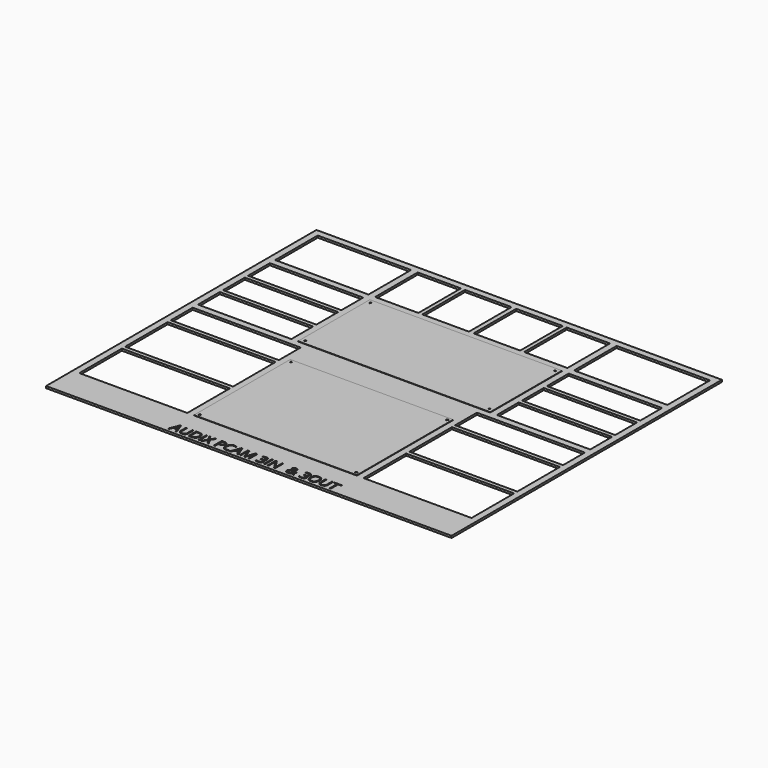
from build123d import *

# Parameters (mm, degrees)
F0_W         = 609.6
F0_H         = 508
F0_W_2       = 162.3
F0_H_2       = 80
F0_H_3       = 41
F0_W_3       = 245
F0_H_4       = 181
F0_W_4       = 140.3
F0_W_5       = 65
F0_W_6       = 70
F0_W_7       = 289
F0_H_5       = 135
F1_DEPTH     = 3
F0_R         = 1.4
F0_W_8       = 269
F0_H_6       = 115
F0_W_9       = 225
F0_H_7       = 161
F2_DEPTH     = 1.5
F3_TEXT_SIZE = 20.8333333333
F4_DEPTH     = 2
F5_SIZE2     = 0.692820323
F5_SIZE      = 0.4
F5_2_SIZE2   = 0.692820323
F5_2_SIZE    = 0.4
F5_3_SIZE2   = 0.692820323
F5_3_SIZE    = 0.4
F5_4_SIZE2   = 0.692820323
F5_4_SIZE    = 0.4
F5_5_SIZE2   = 0.692820323
F5_5_SIZE    = 0.4
F5_6_SIZE2   = 0.692820323
F5_6_SIZE    = 0.4
F5_7_SIZE2   = 0.692820323
F5_7_SIZE    = 0.4
F5_8_SIZE2   = 0.692820323
F5_8_SIZE    = 0.4
F6_START     = 2
F6_DEPTH     = 1.5


# Not quite as in the source:
# - Text() gives the source's letters only with a copy of the font that has no kerning and outlines rounded to 1/6400 em; it was checked with that copy


with BuildPart() as f1:
    # F0 (on Top) → F1 (new body)
    with BuildSketch(Plane.XY):
        Rectangle(F0_W, F0_H)
        with Locations((-213.65, -164)):
            Rectangle(F0_W_2, F0_H_2, mode=Mode.SUBTRACT)
        with Locations((-213.65, -78)):
            Rectangle(F0_W_2, F0_H_2, mode=Mode.SUBTRACT)
        with Locations((-213.65, -11.5)):
            Rectangle(F0_W_2, F0_H_3, mode=Mode.SUBTRACT)
        with Locations((213.65, -164)):
            Rectangle(F0_W_2, F0_H_2, mode=Mode.SUBTRACT)
        with Locations((0, -113.5)):
            Rectangle(F0_W_3, F0_H_4, mode=Mode.SUBTRACT)
        with Locations((213.65, -78)):
            Rectangle(F0_W_2, F0_H_2, mode=Mode.SUBTRACT)
        with Locations((213.65, -11.5)):
            Rectangle(F0_W_2, F0_H_3, mode=Mode.SUBTRACT)
        with Locations((-224.65, 39.5)):
            Rectangle(F0_W_4, F0_H_3, mode=Mode.SUBTRACT)
        with Locations((-224.65, 86.5)):
            Rectangle(F0_W_4, F0_H_3, mode=Mode.SUBTRACT)
        with Locations((-224.65, 133.5)):
            Rectangle(F0_W_4, F0_H_3, mode=Mode.SUBTRACT)
        with Locations((-224.65, 204)):
            Rectangle(F0_W_4, F0_H_2, mode=Mode.SUBTRACT)
        with Locations((-112, 204)):
            Rectangle(F0_W_5, F0_H_2, mode=Mode.SUBTRACT)
        with Locations((-38.5, 204)):
            Rectangle(F0_W_6, F0_H_2, mode=Mode.SUBTRACT)
        with Locations((0, 86.5)):
            Rectangle(F0_W_7, F0_H_5, mode=Mode.SUBTRACT)
        with Locations((224.65, 39.5)):
            Rectangle(F0_W_4, F0_H_3, mode=Mode.SUBTRACT)
        with Locations((224.65, 86.5)):
            Rectangle(F0_W_4, F0_H_3, mode=Mode.SUBTRACT)
        with Locations((38.5, 204)):
            Rectangle(F0_W_6, F0_H_2, mode=Mode.SUBTRACT)
        with Locations((112, 204)):
            Rectangle(F0_W_5, F0_H_2, mode=Mode.SUBTRACT)
        with Locations((224.65, 133.5)):
            Rectangle(F0_W_4, F0_H_3, mode=Mode.SUBTRACT)
        with Locations((224.65, 204)):
            Rectangle(F0_W_4, F0_H_2, mode=Mode.SUBTRACT)
    extrude(amount=F1_DEPTH)



with BuildPart() as f1b:
    # F0 (on Top) → F1, piece 2 (new body)
    with BuildSketch(Plane.XY):
        with Locations((-138.5, 148)):
            Circle(F0_R)
    extrude(amount=F1_DEPTH)


with BuildPart() as f1c:
    # F0 (on Top) → F1, piece 3 (new body)
    with BuildSketch(Plane.XY):
        with Locations((138.5, 148)):
            Circle(F0_R)
    extrude(amount=F1_DEPTH)


with BuildPart() as f1d:
    # F0 (on Top) → F1, piece 4 (new body)
    with BuildSketch(Plane.XY):
        with Locations((138.5, 25)):
            Circle(F0_R)
    extrude(amount=F1_DEPTH)


with BuildPart() as f1e:
    # F0 (on Top) → F1, piece 5 (new body)
    with BuildSketch(Plane.XY):
        with Locations((-138.5, 25)):
            Circle(F0_R)
    extrude(amount=F1_DEPTH)


with BuildPart() as f1f:
    # F0 (on Top) → F1, piece 6 (new body)
    with BuildSketch(Plane.XY):
        with Locations((-117.5, -28)):
            Circle(F0_R)
    extrude(amount=F1_DEPTH)


with BuildPart() as f1g:
    # F0 (on Top) → F1, piece 7 (new body)
    with BuildSketch(Plane.XY):
        with Locations((117.5, -28)):
            Circle(F0_R)
    extrude(amount=F1_DEPTH)


with BuildPart() as f1h:
    # F0 (on Top) → F1, piece 8 (new body)
    with BuildSketch(Plane.XY):
        with Locations((117.5, -199)):
            Circle(F0_R)
    extrude(amount=F1_DEPTH)


with BuildPart() as f1i:
    # F0 (on Top) → F1, piece 9 (new body)
    with BuildSketch(Plane.XY):
        with Locations((-117.5, -199)):
            Circle(F0_R)
    extrude(amount=F1_DEPTH)


with BuildPart() as f1_1:
    add(f1.part)

    add(f1b.part)  # F2 merges F1b

    add(f1c.part)  # F2 merges F1c

    add(f1d.part)  # F2 merges F1d

    add(f1e.part)  # F2 merges F1e

    add(f1f.part)  # F2 merges F1f

    add(f1g.part)  # F2 merges F1g

    add(f1h.part)  # F2 merges F1h

    add(f1i.part)  # F2 merges F1i
    # F0 (on Top) → F2 (join)
    with BuildSketch(Plane.XY):
        with Locations((0, 86.5)):
            Rectangle(F0_W_7, F0_H_5)
        with Locations((-138.5, 25)):
            Circle(F0_R, mode=Mode.SUBTRACT)
        with Locations((-138.5, 148)):
            Circle(F0_R, mode=Mode.SUBTRACT)
        with Locations((138.5, 25)):
            Circle(F0_R, mode=Mode.SUBTRACT)
        with Locations((0, 86.5)):
            Rectangle(F0_W_8, F0_H_6, mode=Mode.SUBTRACT)
        with Locations((138.5, 148)):
            Circle(F0_R, mode=Mode.SUBTRACT)
        with Locations((0, -113.5)):
            Rectangle(F0_W_3, F0_H_4)
        with Locations((-117.5, -199)):
            Circle(F0_R, mode=Mode.SUBTRACT)
        with Locations((-117.5, -28)):
            Circle(F0_R, mode=Mode.SUBTRACT)
        with Locations((117.5, -199)):
            Circle(F0_R, mode=Mode.SUBTRACT)
        with Locations((0, -113.5)):
            Rectangle(F0_W_9, F0_H_7, mode=Mode.SUBTRACT)
        with Locations((117.5, -28)):
            Circle(F0_R, mode=Mode.SUBTRACT)
    extrude(amount=F2_DEPTH)

    # F3 (on face) → F4 (cut)
    with BuildSketch(Plane.XY.offset(3)):
        with Locations((-125.3662109375, -249)):
            Text('AUDIX PCAM 3IN  & 3OUT', F3_TEXT_SIZE, font='Open Sans', text_align=(TextAlign.LEFT, TextAlign.BOTTOM))
    extrude(amount=-F4_DEPTH, mode=Mode.SUBTRACT)

    # F5
    f5_edges = [f1_1.edges().sort_by_distance(p)[0] for p in [
        (-139.9, 148, 3),
    ]]
    f5_side = f1_1.faces().sort_by_distance((-138.5, 148, 3))[0]
    chamfer(f5_edges, length=F5_SIZE, length2=F5_SIZE2, reference=f5_side)

    # F5#2
    f5_2_edges = [f1_1.edges().sort_by_distance(p)[0] for p in [
        (-139.9, 25, 3),
    ]]
    f5_2_side = f1_1.faces().sort_by_distance((-138.5, 25, 3))[0]
    chamfer(f5_2_edges, length=F5_2_SIZE, length2=F5_2_SIZE2, reference=f5_2_side)

    # F5#3
    f5_3_edges = [f1_1.edges().sort_by_distance(p)[0] for p in [
        (137.1, 25, 3),
    ]]
    f5_3_side = f1_1.faces().sort_by_distance((138.5, 25, 3))[0]
    chamfer(f5_3_edges, length=F5_3_SIZE, length2=F5_3_SIZE2, reference=f5_3_side)

    # F5#4
    f5_4_edges = [f1_1.edges().sort_by_distance(p)[0] for p in [
        (137.1, 148, 3),
    ]]
    f5_4_side = f1_1.faces().sort_by_distance((138.5, 148, 3))[0]
    chamfer(f5_4_edges, length=F5_4_SIZE, length2=F5_4_SIZE2, reference=f5_4_side)

    # F5#5
    f5_5_edges = [f1_1.edges().sort_by_distance(p)[0] for p in [
        (116.1, -28, 3),
    ]]
    f5_5_side = f1_1.faces().sort_by_distance((117.5, -28, 3))[0]
    chamfer(f5_5_edges, length=F5_5_SIZE, length2=F5_5_SIZE2, reference=f5_5_side)

    # F5#6
    f5_6_edges = [f1_1.edges().sort_by_distance(p)[0] for p in [
        (-118.9, -28, 3),
    ]]
    f5_6_side = f1_1.faces().sort_by_distance((-117.5, -28, 3))[0]
    chamfer(f5_6_edges, length=F5_6_SIZE, length2=F5_6_SIZE2, reference=f5_6_side)

    # F5#7
    f5_7_edges = [f1_1.edges().sort_by_distance(p)[0] for p in [
        (-118.9, -199, 3),
    ]]
    f5_7_side = f1_1.faces().sort_by_distance((-117.5, -199, 3))[0]
    chamfer(f5_7_edges, length=F5_7_SIZE, length2=F5_7_SIZE2, reference=f5_7_side)

    # F5#8
    f5_8_edges = [f1_1.edges().sort_by_distance(p)[0] for p in [
        (116.1, -199, 3),
    ]]
    f5_8_side = f1_1.faces().sort_by_distance((117.5, -199, 3))[0]
    chamfer(f5_8_edges, length=F5_8_SIZE, length2=F5_8_SIZE2, reference=f5_8_side)


with BuildPart() as f6:
    # F0 (on Top) → F6 (new body)
    with BuildSketch(Plane.XY.offset(F6_START)):
        with Locations((0, 86.5)):
            Rectangle(F0_W_7, F0_H_5)
        with Locations((-138.5, 25)):
            Circle(F0_R, mode=Mode.SUBTRACT)
        with Locations((-138.5, 148)):
            Circle(F0_R, mode=Mode.SUBTRACT)
        with Locations((138.5, 25)):
            Circle(F0_R, mode=Mode.SUBTRACT)
        with Locations((0, 86.5)):
            Rectangle(F0_W_8, F0_H_6, mode=Mode.SUBTRACT)
        with Locations((138.5, 148)):
            Circle(F0_R, mode=Mode.SUBTRACT)
        with Locations((0, 86.5)):
            Rectangle(F0_W_8, F0_H_6)
    extrude(amount=F6_DEPTH)


with BuildPart() as f6b:
    # F0 (on Top) → F6, piece 2 (new body)
    with BuildSketch(Plane.XY.offset(F6_START)):
        with Locations((0, -113.5)):
            Rectangle(F0_W_3, F0_H_4)
        with Locations((-117.5, -199)):
            Circle(F0_R, mode=Mode.SUBTRACT)
        with Locations((-117.5, -28)):
            Circle(F0_R, mode=Mode.SUBTRACT)
        with Locations((117.5, -199)):
            Circle(F0_R, mode=Mode.SUBTRACT)
        with Locations((0, -113.5)):
            Rectangle(F0_W_9, F0_H_7, mode=Mode.SUBTRACT)
        with Locations((117.5, -28)):
            Circle(F0_R, mode=Mode.SUBTRACT)
        with Locations((0, -113.5)):
            Rectangle(F0_W_9, F0_H_7)
    extrude(amount=F6_DEPTH)


solid = Compound([f1_1.part, f6.part, f6b.part])
